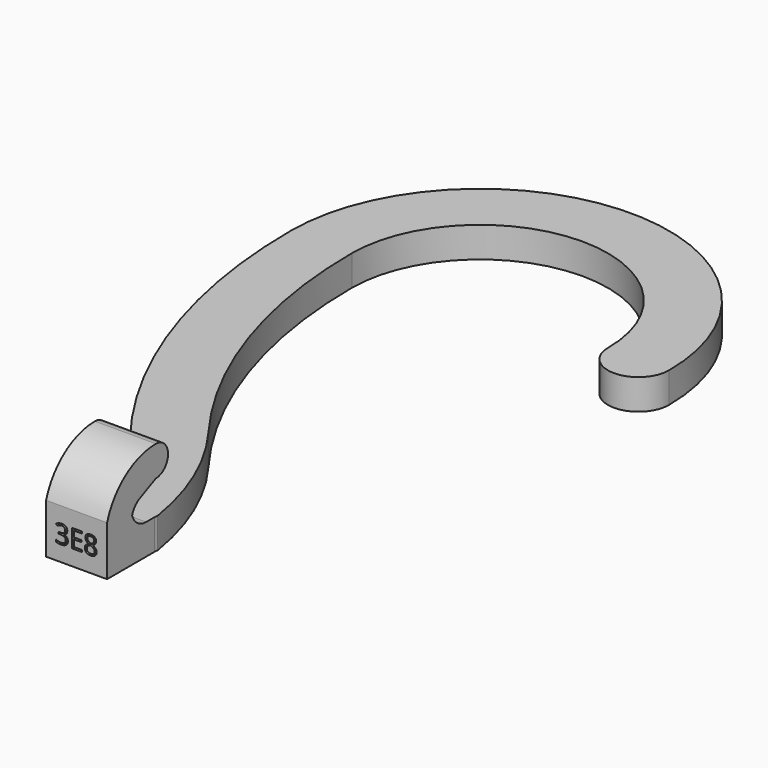
from build123d import *

# Parameters (mm, degrees)
F2_DEPTH     = 5
F4_DEPTH     = 10
F5_TEXT_SIZE = 4.1666666667
F6_DEPTH     = 0.5
F7_T1_DEPTH  = 5
F7_T3_DEPTH  = 10
F8_T1_DEPTH  = 46.9270598238


# Not quite as in the source:
# - a fillet or chamfer that OpenCascade refuses, or shapes differently, is made with other operations: its cross-section is extruded or revolved along the edge and cut away or added
# - Text() gives the source's letters only with a copy of the font that has no kerning and outlines rounded to 1/6400 em; it was checked with that copy


with BuildPart() as f2:
    # F1 (on Top) → F2 (new body)
    with BuildSketch(Plane.XY):
        with BuildLine():
            ThreePointArc((-21, 0), (0, 21), (21, 0))
            ThreePointArc((21, 0), (26, -5), (31, 0))
            ThreePointArc((31, 0), (0, 31), (-31, 0))
            ThreePointArc((-31, 0), (-24.8122094414, -33.5412562826), (-7.0634920635, -62.6666345025))
            Line((-7.0634920635, -62.6666345025), (-5, -72.6666345025))
            Line((-5, -72.6666345025), (-5, -82.6666345025))
            Line((-5, -82.6666345025), (5, -82.6666345025))
            Line((5, -82.6666345025), (5, -72.6666345025))
            Line((5, -72.6666345025), (7.0634920635, -62.6666345025))
            ThreePointArc((7.0634920635, -62.6666345025), (-13.6637680611, -34.3317151722), (-21, 0))
        make_face()
    extrude(amount=F2_DEPTH)

    # F3 (on face) → F4 (join, through all)
    with BuildSketch(Plane.YZ.offset(5)):
        with BuildLine():
            Line((-82.6666345025, 8.1540820259), (-82.6666345025, 5))
            Line((-82.6666345025, 5), (-77.6666345025, 5))
            Line((-77.6666345025, 5), (-77.6666345025, 8.1540820259))
            Line((-77.6666345025, 8.1540820259), (-72.6666345025, 10.4856203167))
            ThreePointArc((-72.6666345025, 10.4856203167), (-70.1666345025, 12.9856203167), (-72.6666345025, 15.4856203167))
            ThreePointArc((-72.6666345025, 15.4856203167), (-78.8664621958, 13.4563804313), (-82.6666345025, 8.1540820259))
        make_face()
    extrude(amount=-F4_DEPTH)

    # F5 (on face) → F6 (cut)
    with BuildSketch(Plane.XZ.offset(82.6666345025)):
        with Locations((-3.5680338542, 2.577041013)):
            Text('3E8', F5_TEXT_SIZE, font='Open Sans', text_align=(TextAlign.LEFT, TextAlign.BOTTOM))
    extrude(amount=-F6_DEPTH, mode=Mode.SUBTRACT)

    # F7: fillet of radius 3 on 5 edges, made by hand

    # F7_s2 → F7_t1 (join)
    with BuildSketch(Plane.XY):
        with BuildLine():
            ThreePointArc((-7.5868858072, -62.0764975819), (-7.1547246678, -62.7193317485), (-6.9015588409, -63.4513878122))
            Line((-6.9015588409, -63.4513878122), (-7.0634920635, -62.6666345025))
            ThreePointArc((-7.0634920635, -62.6666345025), (-7.3258079526, -62.37211505), (-7.5868858072, -62.0764975819))
        make_face()
        with BuildLine():
            ThreePointArc((-5.0619000823, -72.3666571804), (-5.0155151405, -72.6682185842), (-5, -72.9729317666))
            Line((-5, -72.9729317666), (-5, -72.6666345025))
            Line((-5, -72.6666345025), (-5.0619000823, -72.3666571804))
        make_face()
        with BuildLine():
            ThreePointArc((5.0619000823, -72.3666571804), (5.0155151405, -72.6682185842), (5, -72.9729317666))
            Line((5, -72.9729317666), (5, -72.6666345025))
            Line((5, -72.6666345025), (5.0619000823, -72.3666571804))
        make_face()
    extrude(amount=F7_T1_DEPTH)

    # F7_s4 → F7_t3 (join)
    with BuildSketch(Plane.YZ.offset(-5)):
        with BuildLine():
            ThreePointArc((-74.6666345025, 5), (-76.7879548461, 5.8786796564), (-77.6666345025, 8))
            Line((-77.6666345025, 8), (-77.6666345025, 5))
            Line((-77.6666345025, 5), (-74.6666345025, 5))
        make_face()
        with BuildLine():
            ThreePointArc((-77.6666345025, 6.2428712435), (-77.1968088399, 7.8547700686), (-75.9344892877, 8.9617946046))
            Line((-75.9344892877, 8.9617946046), (-77.6666345025, 8.1540820259))
            Line((-77.6666345025, 8.1540820259), (-77.6666345025, 6.2428712435))
        make_face()
    extrude(amount=F7_T3_DEPTH)

    # F8: fillet of radius 50 on 1 edges, made by hand

    # F8_s2 → F8_t1 (cut)
    with BuildSketch(Plane.XY.offset(-41.9270598238)):
        with BuildLine():
            ThreePointArc((-4.2707239758, -50.3055632686), (1.7362268149, -60.7689725472), (5.0619000823, -72.3666571804))
            Line((5.0619000823, -72.3666571804), (7.0634920635, -62.6666345025))
            ThreePointArc((7.0634920635, -62.6666345025), (1.0871215385, -56.769670429), (-4.2707239758, -50.3055632686))
        make_face()
    extrude(amount=F8_T1_DEPTH, mode=Mode.SUBTRACT)


solid = f2.part
